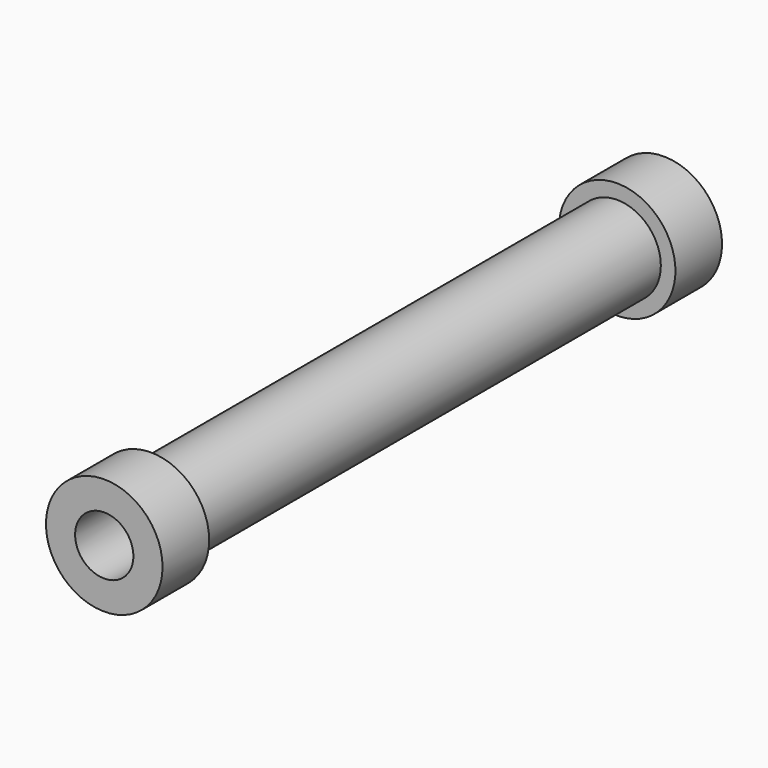
from build123d import *

# Parameters (mm, degrees)
F0_R     = 19.05
F0_R_2   = 15.875
F1_DEPTH = 254
F2_R     = 25.4
F2_R_2   = 6.35
F3_DEPTH = 25.4
F4_R     = 25.4
F4_R_2   = 12.7
F5_DEPTH = 25.4
F7_D     = 12.7
F7_DEPTH = 25.401


with BuildPart() as f1:
    # F0 (on Front) → F1 (new body)
    with BuildSketch(Plane.XZ):
        Circle(F0_R)
        Circle(F0_R_2, mode=Mode.SUBTRACT)
    extrude(amount=F1_DEPTH)

    # F2 (on face) → F3 (join)
    with BuildSketch(Plane(origin=(0, 0, 0), x_dir=(-1, 0, 0), z_dir=(0, 1, 0))):
        Circle(F2_R)
        Circle(F2_R_2, mode=Mode.SUBTRACT)
    extrude(amount=F3_DEPTH)

    # F4 (on face) → F5 (join)
    with BuildSketch(Plane.XZ.offset(254)):
        Circle(F4_R)
        Circle(F4_R_2, mode=Mode.SUBTRACT)
    extrude(amount=F5_DEPTH)

    # F7 (through all, one way)
    with BuildSketch(Plane.YZ):
        with Locations((-228.6, 0)):
            Circle(F7_D / 2)
    extrude(amount=-F7_DEPTH, mode=Mode.SUBTRACT)


solid = f1.part
